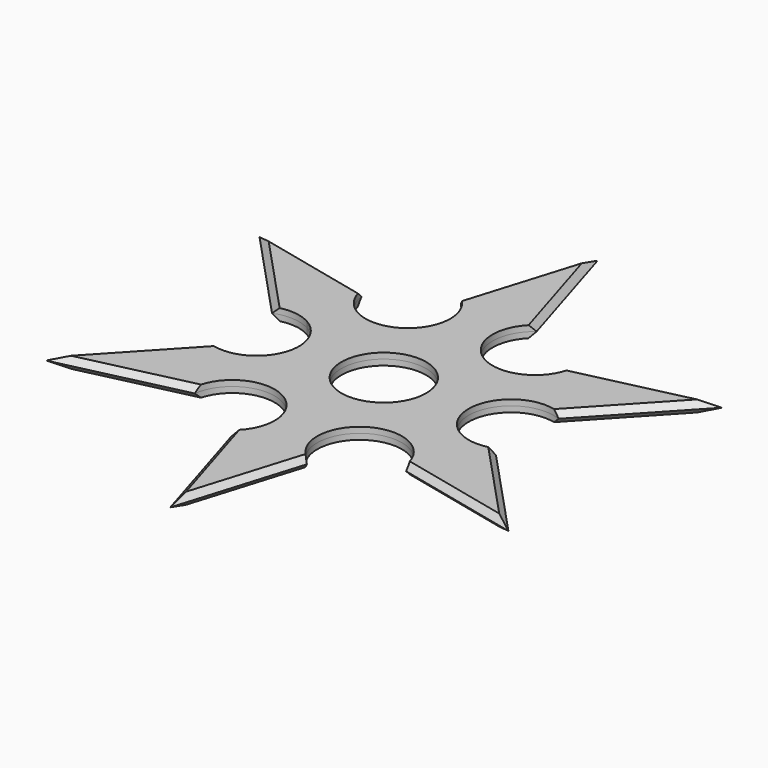
from build123d import *

# Parameters (mm, degrees)
F0_R         = 12.5
F1_DEPTH     = 1.7
F2_T1_DEPTH  = 57.3976375262
F2_T3_DEPTH  = 57.1989693925
F2_T5_DEPTH  = 57.4520267978
F2_T7_DEPTH  = 57.3309437412
F2_T9_DEPTH  = 57.4405501522
F2_T11_DEPTH = 57.3333306688
F2_T13_DEPTH = 57.3176158442
F2_T15_DEPTH = 57.2711320889
F2_T17_DEPTH = 57.4067836399
F2_T19_DEPTH = 57.2939176083
F2_T21_DEPTH = 57.2816108198
F2_T23_DEPTH = 57.2833301593
F3_DEPTH     = 1.7
F4_T1_DEPTH  = 57.4067836399
F4_T3_DEPTH  = 57.2939176083
F4_T5_DEPTH  = 57.2711320889
F4_T7_DEPTH  = 57.3176158442
F4_T9_DEPTH  = 57.3333306688
F4_T11_DEPTH = 57.4405501522
F4_T13_DEPTH = 57.3309437412
F4_T15_DEPTH = 57.4520267978
F4_T17_DEPTH = 57.1989693925
F4_T19_DEPTH = 57.3976375262
F4_T21_DEPTH = 57.2816108198
F4_T23_DEPTH = 57.2833301593


# Not quite as in the source:
# - a fillet or chamfer that OpenCascade refuses, or shapes differently, is made with other operations: its cross-section is extruded or revolved along the edge and cut away or added


with BuildPart() as f1:
    # F0 (on Top) → F1 (new body)
    with BuildSketch(Plane.XY):
        with BuildLine():
            ThreePointArc((-12.6269337533, 21.6838866314), (-18.8533795427, 20.0092263707), (-25.0860923523, 21.6604093381))
            ThreePointArc((-25.0860923523, 21.6604093381), (-29.6261220625, 26.129161021), (-31.3743477244, 32.2549522685))
            Line((-31.3743477244, 32.2549522685), (-72.0726857195, 41.6509039433))
            Line((-72.0726857195, 41.6509039433), (-43.4508925376, 10.9577885101))
            ThreePointArc((-43.4508925376, 10.9577885101), (-37.3541054261, 12.4619159711), (-31.2952509513, 10.8116144975))
            ThreePointArc((-31.2952509513, 10.8116144975), (-26.5801816353, -6.1126428325), (-43.4452596611, -11.0351937982))
            Line((-43.4452596611, -11.0351937982), (-71.9879228197, -41.6434526702))
            Line((-71.9879228197, -41.6434526702), (-31.2073862187, -32.228523952))
            ThreePointArc((-31.2073862187, -32.228523952), (-12.4587232405, -21.6629522163), (-12.2397963262, -43.1826116137))
            Line((-12.2397963262, -43.1826116137), (0, -83.217181477))
            Line((0, -83.217181477), (12.2727951603, -43.0746772909))
            ThreePointArc((12.2727951603, -43.0746772909), (12.5361536488, -21.5848137797), (31.2857724927, -32.0888789276))
            Line((31.2857724927, -32.0888789276), (72.0544236589, -41.501063677))
            Line((72.0544236589, -41.501063677), (43.4872051328, -10.8664723972))
            ThreePointArc((43.4872051328, -10.8664723972), (24.9862322359, 0.0927434014), (43.4764876483, 11.0700319481))
            Line((43.4764876483, 11.0700319481), (72.0544236589, 41.716116323))
            Line((72.0544236589, 41.716116323), (31.1206966034, 32.2658208016))
            ThreePointArc((31.1206966034, 32.2658208016), (12.3360655616, 21.7053334655), (12.2368534674, 43.2547281928))
            Line((12.2368534674, 43.2547281928), (-0.0137682524, 83.324706323))
            Line((-0.0137682524, 83.324706323), (-12.2997912318, 43.1389358899))
            ThreePointArc((-12.2997912318, 43.1389358899), (-7.9575866684, 38.5934345524), (-6.3769337533, 32.5092041787))
            ThreePointArc((-6.3769337533, 32.5092041787), (-8.051616206, 26.2592041787), (-12.6269337533, 21.6838866314))
        make_face()
        Circle(F0_R, mode=Mode.SUBTRACT)
    extrude(amount=F1_DEPTH)

    # F2: chamfer of 3 on 12 edges, made by hand

    # F2_s2 → F2_t1 (cut)
    with BuildSketch(Plane(origin=(-59.5589476137, 63.869151823, 0), x_dir=(0, 0, 1), z_dir=(0.6819983601, -0.7313537016, 0))):
        Polygon((1.7, 21.3047773022), (-1.3, 24.3047773022), (1.7, 24.3047773022), align=None)
    extrude(amount=F2_T1_DEPTH, mode=Mode.SUBTRACT)

    # F2_s4 → F2_t3 (cut)
    with BuildSketch(Plane(origin=(-29.3392197818, 6.7734926001, 0), x_dir=(0, 0, 1), z_dir=(-0.9743700648, 0.2249510543, 0))):
        Polygon((1.7, 21.3705673316), (-1.3, 24.3705673316), (1.7, 24.3705673316), align=None)
    extrude(amount=F2_T3_DEPTH, mode=Mode.SUBTRACT)

    # F2_s6 → F2_t5 (cut)
    with BuildSketch(Plane(origin=(25.5517773205, 83.5760977556, 0), x_dir=(0, 0, 1), z_dir=(-0.2923717047, -0.956304756, 0))):
        Polygon((1.7, 21.3749530784), (-1.3, 24.3749530784), (1.7, 24.3749530784), align=None)
    extrude(amount=F2_T5_DEPTH, mode=Mode.SUBTRACT)

    # F2_s8 → F2_t7 (cut)
    with BuildSketch(Plane(origin=(-8.7921854193, 28.757942701, 0), x_dir=(0, 0, 1), z_dir=(-0.2923717047, 0.956304756, 0))):
        Polygon((1.7, 21.348619788), (-1.3, 24.348619788), (1.7, 24.348619788), align=None)
    extrude(amount=F2_T7_DEPTH, mode=Mode.SUBTRACT)

    # F2_s10 → F2_t9 (cut)
    with BuildSketch(Plane(origin=(85.0691389614, 19.6397582326, 0), x_dir=(0, 0, 1), z_dir=(-0.9743700648, -0.2249510543, 0))):
        Polygon((1.7, 21.438216392), (-1.3, 24.438216392), (1.7, 24.438216392), align=None)
    extrude(amount=F2_T9_DEPTH, mode=Mode.SUBTRACT)

    # F2_s12 → F2_t11 (cut)
    with BuildSketch(Plane(origin=(20.4817428017, 21.9639801073, 0), x_dir=(0, 0, 1), z_dir=(0.6819983601, 0.7313537016, 0))):
        Polygon((1.7, 21.2469465406), (-1.3, 24.2469465406), (1.7, 24.2469465406), align=None)
    extrude(amount=F2_T11_DEPTH, mode=Mode.SUBTRACT)

    # F2_s14 → F2_t13 (cut)
    with BuildSketch(Plane(origin=(59.4757159005, -63.779896738, 0), x_dir=(0, 0, 1), z_dir=(-0.6819983601, 0.7313537016, 0))):
        Polygon((1.7, 21.3936120924), (-1.3, 24.3936120924), (1.7, 24.3936120924), align=None)
    extrude(amount=F2_T13_DEPTH, mode=Mode.SUBTRACT)

    # F2_s16 → F2_t15 (cut)
    with BuildSketch(Plane(origin=(29.2187258401, -6.7456743817, 0), x_dir=(0, 0, 1), z_dir=(0.9743700648, -0.2249510543, 0))):
        Polygon((1.7, 21.2286755314), (-1.3, 24.2286755314), (1.7, 24.2286755314), align=None)
    extrude(amount=F2_T15_DEPTH, mode=Mode.SUBTRACT)

    # F2_s18 → F2_t17 (cut)
    with BuildSketch(Plane(origin=(-25.522890682, -83.4816138184, 0), x_dir=(0, 0, 1), z_dir=(0.2923717047, 0.956304756, 0))):
        Polygon((1.7, 21.3303492106), (-1.3, 24.3303492106), (1.7, 24.3303492106), align=None)
    extrude(amount=F2_T17_DEPTH, mode=Mode.SUBTRACT)

    # F2_s20 → F2_t19 (cut)
    with BuildSketch(Plane(origin=(8.7717703206, -28.6911679218, 0), x_dir=(0, 0, 1), z_dir=(0.2923717047, -0.956304756, 0))):
        Polygon((1.7, 21.3303492106), (-1.3, 24.3303492106), (1.7, 24.3303492106), align=None)
    extrude(amount=F2_T19_DEPTH, mode=Mode.SUBTRACT)

    # F2_s22 → F2_t21 (cut)
    with BuildSketch(Plane(origin=(-20.4498413423, -21.9297699805, 0), x_dir=(0, 0, 1), z_dir=(-0.6819983601, -0.7313537016, 0))):
        Polygon((1.7, 21.2478673976), (-1.3, 24.2478673976), (1.7, 24.2478673976), align=None)
    extrude(amount=F2_T21_DEPTH, mode=Mode.SUBTRACT)

    # F2_s24 → F2_t23 (cut)
    with BuildSketch(Plane(origin=(-84.9900764381, -19.6215052109, 0), x_dir=(0, 0, 1), z_dir=(0.9743700648, 0.2249510543, 0))):
        Polygon((1.7, 21.3823745378), (-1.3, 24.3823745378), (1.7, 24.3823745378), align=None)
    extrude(amount=F2_T23_DEPTH, mode=Mode.SUBTRACT)


with BuildPart() as f3:
    # F0 (on Top) → F3 (new body)
    with BuildSketch(Plane.XY):
        with BuildLine():
            ThreePointArc((-12.640536442, 21.7074471794), (-18.8534308068, 20.0364316999), (-25.072578552, 21.6840209828))
            Line((-25.072578552, 21.6840209828), (-25.0860923523, 21.6604093381))
            ThreePointArc((-25.0860923523, 21.6604093381), (-18.8533795427, 20.0092263707), (-12.6269337533, 21.6838866314))
            Line((-12.6269337533, 21.6838866314), (-12.640536442, 21.7074471794))
        make_face()
        with BuildLine():
            ThreePointArc((-6.4041391307, 32.5092041787), (-8.075176754, 26.2728068674), (-12.640536442, 21.7074471794))
            Line((-12.640536442, 21.7074471794), (-12.6269337533, 21.6838866314))
            ThreePointArc((-12.6269337533, 21.6838866314), (-8.051616206, 26.2592041787), (-6.3769337533, 32.5092041787))
            Line((-6.3769337533, 32.5092041787), (-6.4041391307, 32.5092041787))
        make_face()
        with BuildLine():
            ThreePointArc((-12.6269337533, 21.6838866314), (-18.8533795427, 20.0092263707), (-25.0860923523, 21.6604093381))
            ThreePointArc((-25.0860923523, 21.6604093381), (-29.6261220625, 26.129161021), (-31.3743477244, 32.2549522685))
            Line((-31.3743477244, 32.2549522685), (-72.0726857195, 41.6509039433))
            Line((-72.0726857195, 41.6509039433), (-43.4508925376, 10.9577885101))
            ThreePointArc((-43.4508925376, 10.9577885101), (-37.3541054261, 12.4619159711), (-31.2952509513, 10.8116144975))
            ThreePointArc((-31.2952509513, 10.8116144975), (-26.5801816353, -6.1126428325), (-43.4452596611, -11.0351937982))
            Line((-43.4452596611, -11.0351937982), (-71.9879228197, -41.6434526702))
            Line((-71.9879228197, -41.6434526702), (-31.2073862187, -32.228523952))
            ThreePointArc((-31.2073862187, -32.228523952), (-12.4587232405, -21.6629522163), (-12.2397963262, -43.1826116137))
            Line((-12.2397963262, -43.1826116137), (0, -83.217181477))
            Line((0, -83.217181477), (12.2727951603, -43.0746772909))
            ThreePointArc((12.2727951603, -43.0746772909), (12.5361536488, -21.5848137797), (31.2857724927, -32.0888789276))
            Line((31.2857724927, -32.0888789276), (72.0544236589, -41.501063677))
            Line((72.0544236589, -41.501063677), (43.4872051328, -10.8664723972))
            ThreePointArc((43.4872051328, -10.8664723972), (24.9862322359, 0.0927434014), (43.4764876483, 11.0700319481))
            Line((43.4764876483, 11.0700319481), (72.0544236589, 41.716116323))
            Line((72.0544236589, 41.716116323), (31.1206966034, 32.2658208016))
            ThreePointArc((31.1206966034, 32.2658208016), (12.3360655616, 21.7053334655), (12.2368534674, 43.2547281928))
            Line((12.2368534674, 43.2547281928), (-0.0137682524, 83.324706323))
            Line((-0.0137682524, 83.324706323), (-12.2997912318, 43.1389358899))
            ThreePointArc((-12.2997912318, 43.1389358899), (-7.9575866684, 38.5934345524), (-6.3769337533, 32.5092041787))
            ThreePointArc((-6.3769337533, 32.5092041787), (-8.051616206, 26.2592041787), (-12.6269337533, 21.6838866314))
        make_face()
        Circle(F0_R, mode=Mode.SUBTRACT)
    extrude(amount=-F3_DEPTH)

    # F4: chamfer of 3 on 12 edges, made by hand

    # F4_s2 → F4_t1 (cut)
    with BuildSketch(Plane(origin=(-25.522890682, -83.4816138184, 0), x_dir=(0, 0, 1), z_dir=(0.2923717047, 0.956304756, 0))):
        Polygon((1.3, 24.3303492106), (-1.7, 21.3303492106), (-1.7, 24.3303492106), align=None)
    extrude(amount=F4_T1_DEPTH, mode=Mode.SUBTRACT)

    # F4_s4 → F4_t3 (cut)
    with BuildSketch(Plane(origin=(8.7717703206, -28.6911679218, 0), x_dir=(0, 0, 1), z_dir=(0.2923717047, -0.956304756, 0))):
        Polygon((1.3, 24.3303492106), (-1.7, 21.3303492106), (-1.7, 24.3303492106), align=None)
    extrude(amount=F4_T3_DEPTH, mode=Mode.SUBTRACT)

    # F4_s6 → F4_t5 (cut)
    with BuildSketch(Plane(origin=(29.2187258401, -6.7456743817, 0), x_dir=(0, 0, 1), z_dir=(0.9743700648, -0.2249510543, 0))):
        Polygon((1.3, 24.2286755314), (-1.7, 21.2286755314), (-1.7, 24.2286755314), align=None)
    extrude(amount=F4_T5_DEPTH, mode=Mode.SUBTRACT)

    # F4_s8 → F4_t7 (cut)
    with BuildSketch(Plane(origin=(59.4757159005, -63.779896738, 0), x_dir=(0, 0, 1), z_dir=(-0.6819983601, 0.7313537016, 0))):
        Polygon((1.3, 24.3936120924), (-1.7, 21.3936120924), (-1.7, 24.3936120924), align=None)
    extrude(amount=F4_T7_DEPTH, mode=Mode.SUBTRACT)

    # F4_s10 → F4_t9 (cut)
    with BuildSketch(Plane(origin=(20.4817428017, 21.9639801073, 0), x_dir=(0, 0, 1), z_dir=(0.6819983601, 0.7313537016, 0))):
        Polygon((1.3, 24.2469465406), (-1.7, 21.2469465406), (-1.7, 24.2469465406), align=None)
    extrude(amount=F4_T9_DEPTH, mode=Mode.SUBTRACT)

    # F4_s12 → F4_t11 (cut)
    with BuildSketch(Plane(origin=(85.0691389614, 19.6397582326, 0), x_dir=(0, 0, 1), z_dir=(-0.9743700648, -0.2249510543, 0))):
        Polygon((1.3, 24.438216392), (-1.7, 21.438216392), (-1.7, 24.438216392), align=None)
    extrude(amount=F4_T11_DEPTH, mode=Mode.SUBTRACT)

    # F4_s14 → F4_t13 (cut)
    with BuildSketch(Plane(origin=(-8.7921854193, 28.757942701, 0), x_dir=(0, 0, 1), z_dir=(-0.2923717047, 0.956304756, 0))):
        Polygon((1.3, 24.348619788), (-1.7, 21.348619788), (-1.7, 24.348619788), align=None)
    extrude(amount=F4_T13_DEPTH, mode=Mode.SUBTRACT)

    # F4_s16 → F4_t15 (cut)
    with BuildSketch(Plane(origin=(25.5517773205, 83.5760977556, 0), x_dir=(0, 0, 1), z_dir=(-0.2923717047, -0.956304756, 0))):
        Polygon((1.3, 24.3749530784), (-1.7, 21.3749530784), (-1.7, 24.3749530784), align=None)
    extrude(amount=F4_T15_DEPTH, mode=Mode.SUBTRACT)

    # F4_s18 → F4_t17 (cut)
    with BuildSketch(Plane(origin=(-29.3392197818, 6.7734926001, 0), x_dir=(0, 0, 1), z_dir=(-0.9743700648, 0.2249510543, 0))):
        Polygon((1.3, 24.3705673316), (-1.7, 21.3705673316), (-1.7, 24.3705673316), align=None)
    extrude(amount=F4_T17_DEPTH, mode=Mode.SUBTRACT)

    # F4_s20 → F4_t19 (cut)
    with BuildSketch(Plane(origin=(-59.5589476137, 63.869151823, 0), x_dir=(0, 0, 1), z_dir=(0.6819983601, -0.7313537016, 0))):
        Polygon((1.3, 24.3047773022), (-1.7, 21.3047773022), (-1.7, 24.3047773022), align=None)
    extrude(amount=F4_T19_DEPTH, mode=Mode.SUBTRACT)

    # F4_s22 → F4_t21 (cut)
    with BuildSketch(Plane(origin=(-20.4498413423, -21.9297699805, 0), x_dir=(0, 0, 1), z_dir=(-0.6819983601, -0.7313537016, 0))):
        Polygon((1.3, 24.2478673976), (-1.7, 21.2478673976), (-1.7, 24.2478673976), align=None)
    extrude(amount=F4_T21_DEPTH, mode=Mode.SUBTRACT)

    # F4_s24 → F4_t23 (cut)
    with BuildSketch(Plane(origin=(-84.9900764381, -19.6215052109, 0), x_dir=(0, 0, 1), z_dir=(0.9743700648, 0.2249510543, 0))):
        Polygon((1.3, 24.3823745378), (-1.7, 21.3823745378), (-1.7, 24.3823745378), align=None)
    extrude(amount=F4_T23_DEPTH, mode=Mode.SUBTRACT)


solid = Compound([f1.part, f3.part])
